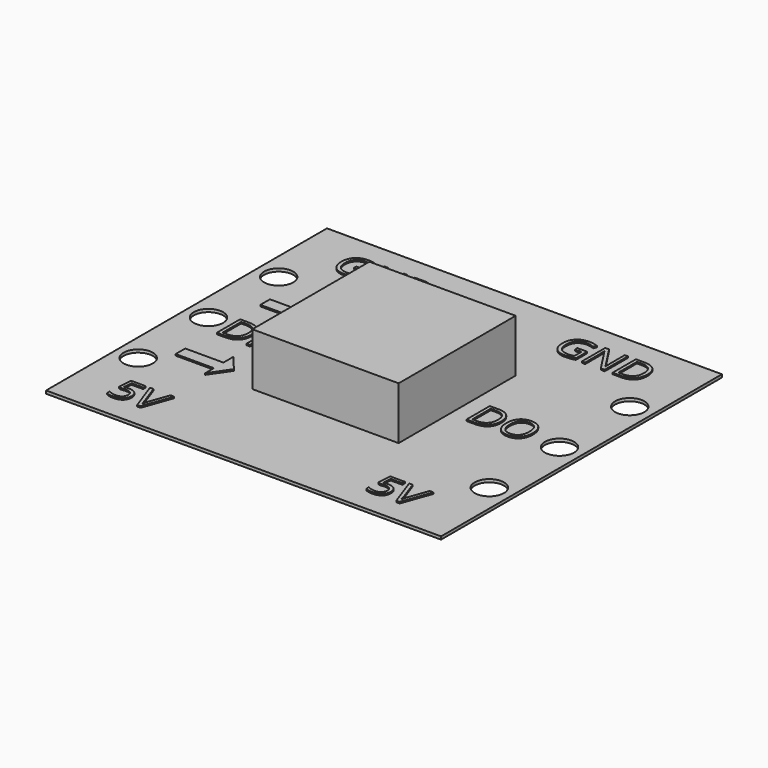
from build123d import *

# Parameters (mm, degrees)
F0_W         = 13.5
F0_H         = 12
F0_R         = 0.5
F1_DEPTH     = 0.1
F2_W         = 5
F2_H         = 5
F3_DEPTH     = 1.8
F4_TEXT_SIZE = 1.3888888889
F5_DEPTH     = 0.05


# Not quite as in the source:
# - Text() gives the source's letters only with a copy of the font that has no kerning and outlines rounded to 1/6400 em; it was checked with that copy


with BuildPart() as f1:
    # F0 (on Top) → F1 (new body)
    with BuildSketch(Plane.XY):
        Rectangle(F0_W, F0_H)
        with Locations((-6, -3)):
            Circle(F0_R, mode=Mode.SUBTRACT)
        with Locations((6, -3)):
            Circle(F0_R, mode=Mode.SUBTRACT)
        with Locations((-6, 0)):
            Circle(F0_R, mode=Mode.SUBTRACT)
        with Locations((-6, 3)):
            Circle(F0_R, mode=Mode.SUBTRACT)
        with Locations((6, 0)):
            Circle(F0_R, mode=Mode.SUBTRACT)
        with Locations((6, 3)):
            Circle(F0_R, mode=Mode.SUBTRACT)
    extrude(amount=F1_DEPTH)

    # F2 (on face) → F3 (join)
    with BuildSketch(Plane.XY.offset(0.1)):
        Rectangle(F2_W, F2_H)
    extrude(amount=F3_DEPTH)

    # F4 (on face) → F5 (join)
    with BuildSketch(Plane.XY.offset(0.1)):
        Polygon((-4.01157327, 1.7719101161), (-5.3151287138, 1.7719101161), (-5.3151287138, 1.3622213155), (-4.01157327, 1.3622213155), (-4.0093539283, 1.3135385234), (-4.005968105, 0.9877872653), (-3.5555742215, 1.6489408445), (-4.01157327, 2.2013681009), align=None)
        Polygon((-4.0009262448, -1.8605308724), (-5.3044816887, -1.8605308724), (-5.3044816887, -2.2702196729), (-4.0009262448, -2.2702196729), (-3.9987069031, -2.318902465), (-3.9953210799, -2.6446537231), (-3.5449271963, -1.983500144), (-4.0009262448, -1.4310728875), align=None)
        with Locations((-5.2720677258, 4.1734123513)):
            Text('GND', F4_TEXT_SIZE, font='Open Sans', text_align=(TextAlign.LEFT, TextAlign.BOTTOM))
        with Locations((-5.3519061382, -0.6192143203)):
            Text('DI', F4_TEXT_SIZE, font='Open Sans', text_align=(TextAlign.LEFT, TextAlign.BOTTOM))
        with Locations((-5.4183909527, -5.2095681889)):
            Text('5V', F4_TEXT_SIZE, font='Open Sans', text_align=(TextAlign.LEFT, TextAlign.BOTTOM))
        with Locations((2.2807543947, 4.176211907)):
            Text('GND', F4_TEXT_SIZE, font='Open Sans', text_align=(TextAlign.LEFT, TextAlign.BOTTOM))
        with Locations((3.4379862625, -5.2067685169)):
            Text('5V', F4_TEXT_SIZE, font='Open Sans', text_align=(TextAlign.LEFT, TextAlign.BOTTOM))
        with Locations((2.9833680019, -0.3722804502)):
            Text('DO', F4_TEXT_SIZE, font='Open Sans', text_align=(TextAlign.LEFT, TextAlign.BOTTOM))
    extrude(amount=F5_DEPTH)


solid = f1.part
